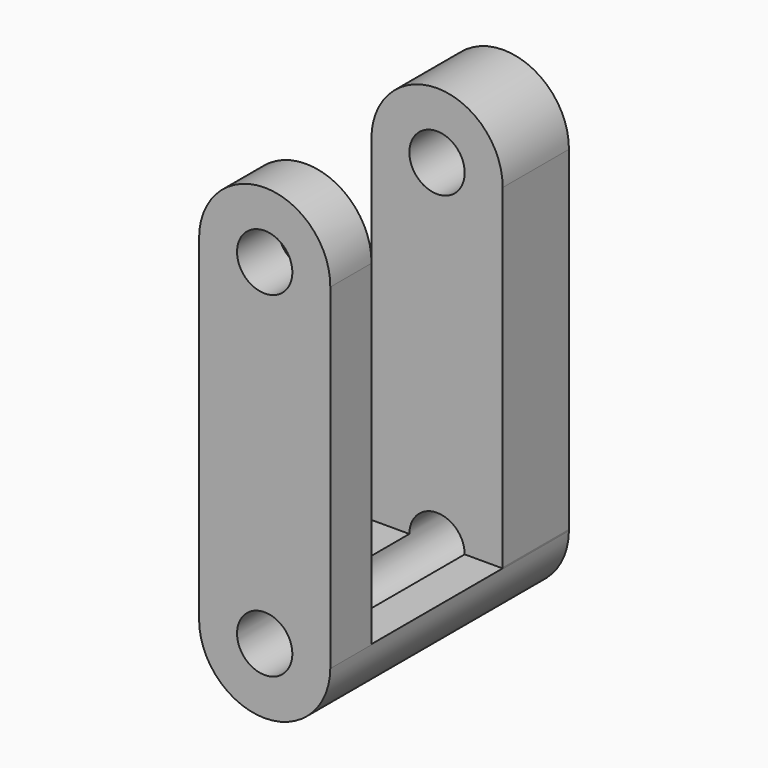
from build123d import *

# Parameters (mm, degrees)
F0_R     = 8.4832662773
F1_DEPTH = 91.44
F2_W     = 59.8430555439
F2_H     = 102.967698127
F3_DEPTH = 57.658
F4_DEPTH = 25.4


# Not quite as in the source:
# - the program builds the solid bodies; features that only make, move or delete a surface that nothing else refers to are left out


with BuildPart() as f1:
    # F0 (on Front) → F1 (new body)
    with BuildSketch(Plane.XZ):
        with BuildLine():
            Line((20.1094433592, -48.163229742), (20.1094433592, 54.4155371868))
            ThreePointArc((20.1094433592, 54.4155371868), (0.0972339361, 74.7201513345), (-20.1103836136, 54.6100027859))
            Line((-20.1103836136, 54.6100027859), (-20.1103836136, -48.3576953411))
            ThreePointArc((-20.1103836136, -48.3576953411), (-0.0972339361, -28.2475467925), (20.1094433592, -48.163229742))
        make_face()
        with Locations((0, 54.6100027859)):
            Circle(F0_R, mode=Mode.SUBTRACT)
        with BuildLine():
            Line((20.1094433592, -48.5521609402), (20.1094433592, -48.163229742))
            ThreePointArc((20.1094433592, -48.163229742), (-0.0972339361, -28.2475467925), (-20.1103836136, -48.3576953411))
            ThreePointArc((-20.1103836136, -48.3576953411), (-0.0972339361, -68.4678438897), (20.1094433592, -48.5521609402))
        make_face()
        with Locations((0, -48.3576953411)):
            Circle(F0_R, mode=Mode.SUBTRACT)
    extrude(amount=F1_DEPTH)

    # F2 (on face) → F3 (cut)
    with BuildSketch(Plane(origin=(-20.1103836136, 0, 0), x_dir=(0, -1, 0), z_dir=(-1, 0, 0))):
        with Locations((45.72, 106.0938518494)):
            Rectangle(F2_W, F2_H)
        with Locations((45.72, 3.1261537224)):
            Rectangle(F2_W, F2_H)
    extrude(amount=-F3_DEPTH, mode=Mode.SUBTRACT)

    # F0 (on Front) → F4 (join)
    with BuildSketch(Plane.XZ):
        with BuildLine():
            Line((20.1094433592, -48.163229742), (20.1094433592, 54.4155371868))
            ThreePointArc((20.1094433592, 54.4155371868), (0.0972339361, 74.7201513345), (-20.1103836136, 54.6100027859))
            Line((-20.1103836136, 54.6100027859), (-20.1103836136, -48.3576953411))
            ThreePointArc((-20.1103836136, -48.3576953411), (-0.0972339361, -28.2475467925), (20.1094433592, -48.163229742))
        make_face()
        with Locations((0, 54.6100027859)):
            Circle(F0_R, mode=Mode.SUBTRACT)
        with BuildLine():
            Line((20.1094433592, -48.5521609402), (20.1094433592, -48.163229742))
            ThreePointArc((20.1094433592, -48.163229742), (-0.0972339361, -28.2475467925), (-20.1103836136, -48.3576953411))
            ThreePointArc((-20.1103836136, -48.3576953411), (-0.0972339361, -68.4678438897), (20.1094433592, -48.5521609402))
        make_face()
        with Locations((0, -48.3576953411)):
            Circle(F0_R, mode=Mode.SUBTRACT)
        with BuildLine():
            ThreePointArc((20.1103836136, -48.3576953411), (20.1101485486, -48.260461405), (20.1094433592, -48.163229742))
            Line((20.1094433592, -48.163229742), (20.1094433592, -48.5521609402))
            ThreePointArc((20.1094433592, -48.5521609402), (20.1101485486, -48.4549292772), (20.1103836136, -48.3576953411))
        make_face()
    extrude(amount=F4_DEPTH)


solid = f1.part
